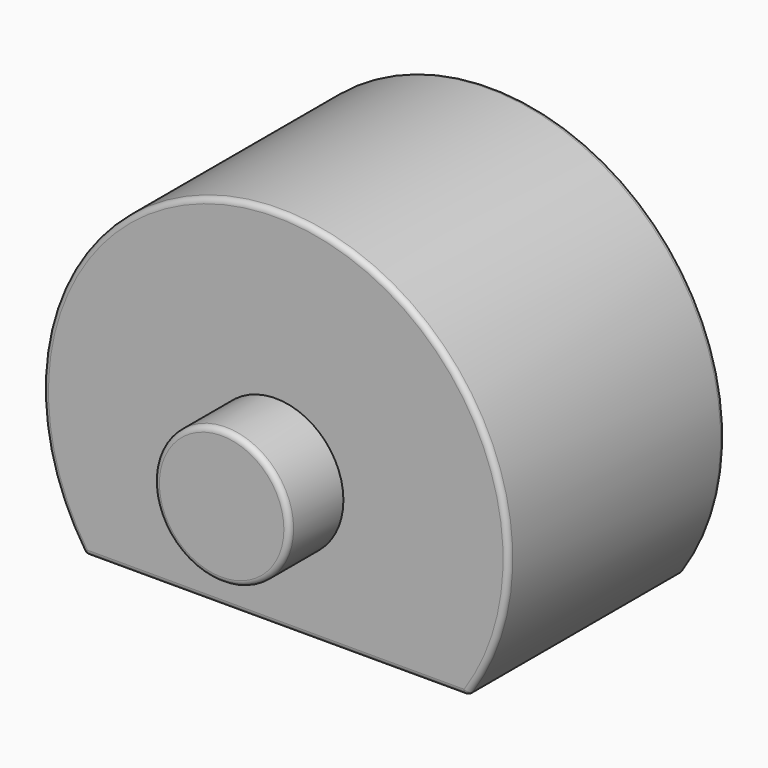
from build123d import *

# Parameters (mm, degrees)
F3_DEPTH = 6.35
F1_R     = 3.175
F4_DEPTH = 9.525
F2_R     = 3.175
F5_DEPTH = 12.7
F6_R     = 0.254


with BuildPart() as f3:
    # F0 (on Front) → F3 (new body, symmetric)
    with BuildSketch(Plane.XZ):
        with BuildLine():
            Line((-8.9757648699, 0), (8.9757648699, 0))
            ThreePointArc((8.9757648699, 0), (0, 17.145), (-8.9757648699, 0))
        make_face()
    extrude(amount=F3_DEPTH, both=True)

    # F1 (on Front) → F4 (join, symmetric)
    with BuildSketch(Plane.XZ):
        with Locations((0, 6.223)):
            Circle(F1_R)
    extrude(amount=F4_DEPTH, both=True)

    # F2 (on Top) → F5 (cut)
    with BuildSketch(Plane.XY):
        Circle(F2_R)
    extrude(amount=F5_DEPTH, mode=Mode.SUBTRACT)

    # F6
    f6_edges = [f3.edges().sort_by_distance(p)[0] for p in [
        (0, -6.35, 17.145),
        (0, 6.35, 17.145),
        (8.975765, 0, 0),
        (0, -6.35, 0),
        (-3.175, -9.525, 6.223),
        (0, 6.35, 0),
        (-8.975765, 0, 0),
    ]]
    fillet(f6_edges, radius=F6_R)


solid = f3.part
